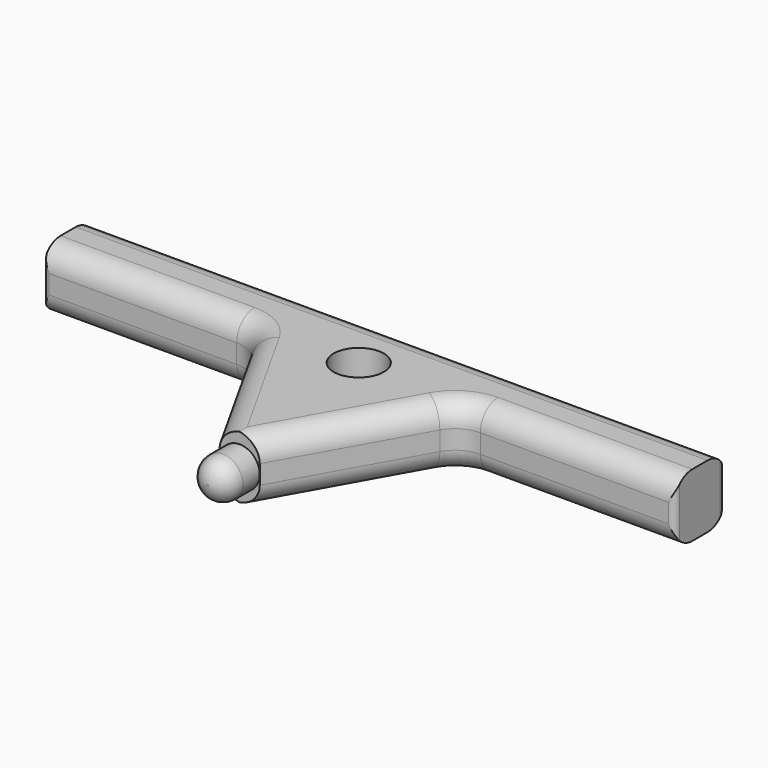
from build123d import *

# Parameters (mm, degrees)
F0_R         = 7.935
F1_DEPTH     = 20
F2_DEPTH     = 12.7
F4_DEPTH     = 12.7
F6_T1_DEPTH  = 77.0257979591
F6_T3_DEPTH  = 76.8715237662
F6_T5_DEPTH  = 231
F6_T8_ANGLE  = 60.7302478015
F6_T12_DEPTH = 65.5200608313
F6_T17_DEPTH = 65.5200608313
F6_T20_ANGLE = 60.7302478015
F6_T22_ANGLE = 60.7302478015
F6_T26_DEPTH = 65.5200608313
F6_T31_DEPTH = 65.5200608313
F6_T34_ANGLE = 60.7302478015


# Not quite as in the source:
# - a fillet or chamfer that OpenCascade refuses, or shapes differently, is made with other operations: its cross-section is extruded or revolved along the edge and cut away or added


with BuildPart() as f1:
    # F0 (on Top) → F1 (new body)
    with BuildSketch(Plane.XY):
        with BuildLine():
            Line((98, 20), (-98, 20))
            ThreePointArc((-98, 20), (-99.4142135624, 19.4142135624), (-100, 18))
            Line((-100, 18), (-100, 2))
            ThreePointArc((-100, 2), (-99.4142135624, 0.5857864376), (-98, 0))
            Line((-98, 0), (-38.6284762338, 0))
            ThreePointArc((-38.6284762338, 0), (-33.5733896743, -1.3717846645), (-29.9052011587, -5.1107800249))
            Line((-29.9052011587, -5.1107800249), (-6.4271370964, -47))
            Line((-6.4271370964, -47), (-6.4271370964, -59.7))
            Line((-6.4271370964, -59.7), (6.2728629036, -59.7))
            Line((6.2728629036, -59.7), (6.2728629036, -47))
            Line((6.2728629036, -47), (29.7509269659, -5.1107800249))
            ThreePointArc((29.7509269659, -5.1107800249), (33.4191154814, -1.3717846645), (38.4742020409, 0))
            Line((38.4742020409, 0), (98, 0))
            ThreePointArc((98, 0), (99.4142135624, 0.5857864376), (100, 2))
            Line((100, 2), (100, 18))
            ThreePointArc((100, 18), (99.4142135624, 19.4142135624), (98, 20))
        make_face()
        Circle(F0_R, mode=Mode.SUBTRACT)
    extrude(amount=F1_DEPTH)

    # F2 (cut): a face of the model
    f2_faces = [f1.faces().sort_by_distance(p)[0] for p in [
        (-0.0771370964, -59.7, 10),
    ]]
    extrude(f2_faces, amount=-F2_DEPTH, mode=Mode.SUBTRACT)

    # F3 (on face) → F4 (join)
    with BuildSketch(Plane.XZ.offset(47)):
        with BuildLine():
            ThreePointArc((-6.4271370964, 10), (-0.0771370964, 3.65), (6.2728629036, 10))
            ThreePointArc((6.2728629036, 10), (-0.0771370964, 16.35), (-6.4271370964, 10))
        make_face()
    extrude(amount=F4_DEPTH)

    # F5: fillet of radius 6.0355339059 on 1 edges, made by hand

    # F5_s1 → F5_t2 (revolve, cut)
    with BuildSketch(Plane.XY.offset(10)):
        with BuildLine():
            ThreePointArc((-6.4271370964, -53.6644660941), (-4.6593701435, -57.932233047), (-0.3916031905, -59.7))
            Line((-0.3916031905, -59.7), (-6.4271370964, -59.7))
            Line((-6.4271370964, -59.7), (-6.4271370964, -53.6644660941))
        make_face()
    revolve(axis=Axis((-0.0771370964, -59.7, 10), (0, 1, 0)), mode=Mode.SUBTRACT)

    # F6: fillet of radius 7 on 14 edges, made by hand

    # F6_s2 → F6_t1 (cut)
    with BuildSketch(Plane.YZ.offset(38.4742020409)):
        with BuildLine():
            ThreePointArc((7, 0), (2.0502525317, 2.0502525317), (0, 7))
            Line((0, 7), (0, 0))
            Line((0, 0), (7, 0))
        make_face()
        with BuildLine():
            ThreePointArc((7, 20), (2.0502525317, 17.9497474683), (0, 13))
            Line((0, 13), (0, 20))
            Line((0, 20), (7, 20))
        make_face()
    extrude(amount=F6_T1_DEPTH, mode=Mode.SUBTRACT)

    # F6_s4 → F6_t3 (cut)
    with BuildSketch(Plane.YZ.offset(-115.5)):
        with BuildLine():
            ThreePointArc((7, 0), (2.0502525317, 2.0502525317), (0, 7))
            Line((0, 7), (0, 0))
            Line((0, 0), (7, 0))
        make_face()
        with BuildLine():
            ThreePointArc((7, 20), (2.0502525317, 17.9497474683), (0, 13))
            Line((0, 13), (0, 20))
            Line((0, 20), (7, 20))
        make_face()
    extrude(amount=F6_T3_DEPTH, mode=Mode.SUBTRACT)

    # F6_s6 → F6_t5 (cut)
    with BuildSketch(Plane.YZ.offset(-115.5)):
        with BuildLine():
            ThreePointArc((13, 0), (17.9497474683, 2.0502525317), (20, 7))
            Line((20, 7), (20, 0))
            Line((20, 0), (13, 0))
        make_face()
        with BuildLine():
            ThreePointArc((13, 20), (17.9497474683, 17.9497474683), (20, 13))
            Line((20, 13), (20, 20))
            Line((20, 20), (13, 20))
        make_face()
    extrude(amount=F6_T5_DEPTH, mode=Mode.SUBTRACT)

    # F6_s7 → F6_t8 (revolve, cut)
    with BuildSketch(Plane(origin=(4.9320537662, 8.7996985012, 0), x_dir=(0, 0, 1), z_dir=(-0.4889219975, -0.8723275075, 0))):
        with BuildLine():
            ThreePointArc((0, -21.4513247447), (2.0502525317, -26.401072213), (7, -28.4513247447))
            Line((7, -28.4513247447), (0, -28.4513247447))
            Line((0, -28.4513247447), (0, -21.4513247447))
        make_face()
    revolve(axis=Axis((38.4742020409, -10, 0), (0, 0, -1)), revolution_arc=F6_T8_ANGLE, mode=Mode.SUBTRACT)


with BuildPart() as f6_tool10:
    # F6_s11 → F6_t12 (new body)
    with BuildSketch(Plane(origin=(-27.1021452526, -48.3552528553, 0), x_dir=(0, 0, 1), z_dir=(0.4889219975, 0.8723275075, 0))):
        with BuildLine():
            ThreePointArc((7, 28.4513247447), (2.0502525317, 26.401072213), (0, 21.4513247447))
            Line((0, 21.4513247447), (0, 28.4513247447))
            Line((0, 28.4513247447), (7, 28.4513247447))
        make_face()
    extrude(amount=F6_T12_DEPTH)

    split(bisect_by=Plane.XZ.offset(47), keep=Keep.BOTTOM)


with BuildPart() as f1_1:
    add(f1.part)

    # F6_t9: cut F6_tool10
    add(f6_tool10.part, mode=Mode.SUBTRACT)


with BuildPart() as f6_tool15:
    # F6_s16 → F6_t17 (new body)
    with BuildSketch(Plane(origin=(-4.9689321973, 8.865496461, 0), x_dir=(0, 0, 1), z_dir=(0.4889219975, -0.8723275075, 0))):
        with BuildLine():
            ThreePointArc((7, 28.5859023668), (2.0502525317, 26.5356498351), (0, 21.5859023668))
            Line((0, 21.5859023668), (0, 28.5859023668))
            Line((0, 28.5859023668), (7, 28.5859023668))
        make_face()
    extrude(amount=F6_T17_DEPTH)

    split(bisect_by=Plane.XZ.offset(47), keep=Keep.BOTTOM)


with BuildPart() as f1_2:
    add(f1_1.part)

    # F6_t14: cut F6_tool15
    add(f6_tool15.part, mode=Mode.SUBTRACT)

    # F6_s19 → F6_t20 (revolve, cut)
    with BuildSketch(Plane.YZ.offset(-38.6284762338)):
        with BuildLine():
            ThreePointArc((7, 0), (2.0502525317, 2.0502525317), (0, 7))
            Line((0, 7), (0, 0))
            Line((0, 0), (7, 0))
        make_face()
    revolve(axis=Axis((-38.6284762338, -10, 0), (0, 0, -1)), revolution_arc=F6_T20_ANGLE, mode=Mode.SUBTRACT)

    # F6_s21 → F6_t22 (revolve, cut)
    with BuildSketch(Plane(origin=(4.9320537662, 8.7996985012, 0), x_dir=(0, 0, 1), z_dir=(-0.4889219975, -0.8723275075, 0))):
        with BuildLine():
            ThreePointArc((20, -21.4513247447), (17.9497474683, -26.401072213), (13, -28.4513247447))
            Line((13, -28.4513247447), (20, -28.4513247447))
            Line((20, -28.4513247447), (20, -21.4513247447))
        make_face()
    revolve(axis=Axis((38.4742020409, -10, 20), (0, 0, -1)), revolution_arc=F6_T22_ANGLE, mode=Mode.SUBTRACT)


with BuildPart() as f6_tool24:
    # F6_s25 → F6_t26 (new body)
    with BuildSketch(Plane(origin=(-27.1021452526, -48.3552528553, 0), x_dir=(0, 0, 1), z_dir=(0.4889219975, 0.8723275075, 0))):
        with BuildLine():
            ThreePointArc((13, 28.4513247447), (17.9497474683, 26.401072213), (20, 21.4513247447))
            Line((20, 21.4513247447), (20, 28.4513247447))
            Line((20, 28.4513247447), (13, 28.4513247447))
        make_face()
    extrude(amount=F6_T26_DEPTH)

    split(bisect_by=Plane.XZ.offset(47), keep=Keep.BOTTOM)


with BuildPart() as f1_3:
    add(f1_2.part)

    # F6_t23: cut F6_tool24
    add(f6_tool24.part, mode=Mode.SUBTRACT)


with BuildPart() as f6_tool29:
    # F6_s30 → F6_t31 (new body)
    with BuildSketch(Plane(origin=(-4.9689321973, 8.865496461, 0), x_dir=(0, 0, 1), z_dir=(0.4889219975, -0.8723275075, 0))):
        with BuildLine():
            ThreePointArc((20, 21.5859023668), (17.9497474683, 26.5356498351), (13, 28.5859023668))
            Line((13, 28.5859023668), (20, 28.5859023668))
            Line((20, 28.5859023668), (20, 21.5859023668))
        make_face()
    extrude(amount=F6_T31_DEPTH)

    split(bisect_by=Plane.XZ.offset(47), keep=Keep.BOTTOM)


with BuildPart() as f1_4:
    add(f1_3.part)

    # F6_t28: cut F6_tool29
    add(f6_tool29.part, mode=Mode.SUBTRACT)

    # F6_s33 → F6_t34 (revolve, cut)
    with BuildSketch(Plane.YZ.offset(-38.6284762338)):
        with BuildLine():
            ThreePointArc((7, 20), (2.0502525317, 17.9497474683), (0, 13))
            Line((0, 13), (0, 20))
            Line((0, 20), (7, 20))
        make_face()
    revolve(axis=Axis((-38.6284762338, -10, 20), (0, 0, -1)), revolution_arc=F6_T34_ANGLE, mode=Mode.SUBTRACT)


solid = f1_4.part
